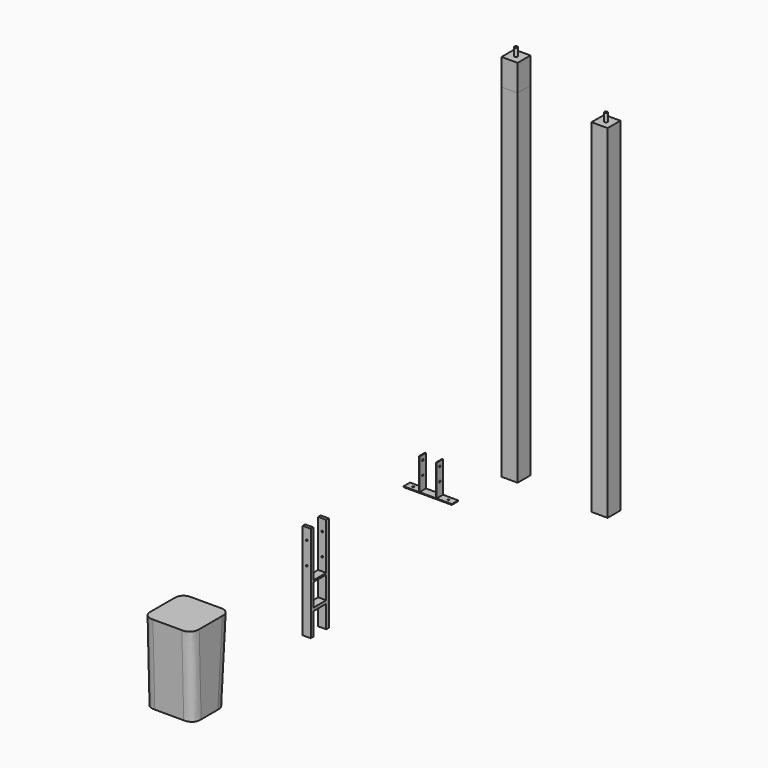
from build123d import *

# Parameters (mm, degrees)
F0_W         = 100
F0_H         = 100
F1_DEPTH     = 2300
F2_DEPTH     = 2135
F3_R         = 10
F4_DEPTH     = 50
F5_R         = 10
F6_DEPTH     = 50
F7_W         = 140
F7_H         = 600
F8_DEPTH     = 50
F9_W         = 101
F9_H         = 290.5959367752
F9_H_2       = 140
F10_DEPTH    = 100.001
F11_DEPTH    = 300
F12_T1_DEPTH = 800.2260480622
F12_T3_DEPTH = 801.2209490406
F14_W        = 300
F14_H        = 50
F15_DEPTH    = 200
F16_W        = 94.5
F16_H        = 195
F16_W_2      = 101
F17_DEPTH    = 482.3491559753
F19_D        = 10.5
F20_D        = 10.5
F21_D        = 10.5


# Not quite as in the source:
# - a fillet or chamfer that OpenCascade refuses, or shapes differently, is made with other operations: its cross-section is extruded or revolved along the edge and cut away or added


with BuildPart() as f1:
    # F0 (on Top) → F1 (new body)
    with BuildSketch(Plane.XY):
        Rectangle(F0_W, F0_H)
    extrude(amount=F1_DEPTH)

    # F3 (on face) → F4 (join)
    with BuildSketch(Plane.XY.offset(2300)):
        Circle(F3_R)
    extrude(amount=F4_DEPTH)


with BuildPart() as f2:
    # F0 (on Top) → F2 (new body)
    with BuildSketch(Plane.XY):
        Rectangle(F0_W, F0_H)
    extrude(amount=F2_DEPTH)


with BuildPart() as f2b:
    # F0 (on Top) → F2, piece 2 (new body)
    with BuildSketch(Plane.XY):
        with Locations((572.3989486694, -15.5273422599)):
            Rectangle(F0_W, F0_H)
    extrude(amount=F2_DEPTH)

    # F5 (on face) → F6 (join)
    with BuildSketch(Plane.XY.offset(2135)):
        with Locations((572.3989486694, -15.5273422599)):
            Circle(F5_R)
    extrude(amount=F6_DEPTH)


with BuildPart() as f8:
    # F7 (on Right) → F8 (new body)
    with BuildSketch(Plane.YZ):
        with Locations((-1588.707132116, 102.0108014345)):
            Rectangle(F7_W, F7_H)
    extrude(amount=F8_DEPTH)

    # F9 (on face) → F10 (cut, through all)
    with BuildSketch(Plane.YZ.offset(50)):
        with Locations((-1588.707132116, 256.7128330469)):
            Rectangle(F9_W, F9_H)
        with Locations((-1588.707132116, 31.4230661094)):
            Rectangle(F9_W, F9_H_2)
        with Locations((-1588.707132116, -127.9891985655)):
            Rectangle(F9_W, F9_H_2)
    extrude(amount=-F10_DEPTH, mode=Mode.SUBTRACT)

    # F19 (through all)
    with Locations(Plane.XZ.offset(1658.707132116)):
        with Locations((25, 330.6745588779), (25, 191.4181262255)):
            Hole(F19_D / 2)


with BuildPart() as f11:
    # F9 (on face) → F11 (new body)
    with BuildSketch(Plane.YZ.offset(50)):
        Polygon((-2661.4876322974, 454.1331665205), (-2961.4876322974, 454.1331665205), (-2946.4510382692, -45.8668334795), (-2696.4510382692, -45.8668334795), align=None)
    extrude(amount=F11_DEPTH)

    # F12: fillet of radius 60 on 4 edges, made by hand

    # F12_s2 → F12_t1 (cut)
    with BuildSketch(Plane(origin=(0, -20.8297708127, 692.6359378174), x_dir=(1, 0, 0), z_dir=(0, 0.0300595982, -0.9995481082))):
        with BuildLine():
            add(Edge.make_bspline(
                [(290, 2946.4982997158), (350, 2946.4982997158), (350, 2886.4982997158)],
                knots=[0, 0, 0, 1, 1, 1], degree=2, weights=[1, 1, 1]))
            Line((350, 2886.4982997158), (350, 2946.4982997158))
            Line((350, 2946.4982997158), (290, 2946.4982997158))
        make_face()
        with BuildLine():
            add(Edge.make_bspline(
                [(110, 2946.4982997158), (50, 2946.4982997158), (50, 2886.4982997158)],
                knots=[0, 0, 0, 1, 1, 1], degree=2, weights=[1, 1, 1]))
            Line((50, 2886.4982997158), (50, 2946.4982997158))
            Line((50, 2946.4982997158), (110, 2946.4982997158))
        make_face()
    extrude(amount=F12_T1_DEPTH, mode=Mode.SUBTRACT)

    # F12_s4 → F12_t3 (cut)
    with BuildSketch(Plane(origin=(0, -26.776023858, -382.9149808747), x_dir=(1, 0, 0), z_dir=(0, 0.0697564737, 0.9975640503))):
        with BuildLine():
            add(Edge.make_bspline(
                [(110, -2686.6831104978), (50, -2686.6831104978), (50, -2746.6831104978)],
                knots=[0, 0, 0, 1, 1, 1], degree=2, weights=[1, 1, 1]))
            Line((50, -2746.6831104978), (50, -2686.6831104978))
            Line((50, -2686.6831104978), (110, -2686.6831104978))
        make_face()
        with BuildLine():
            add(Edge.make_bspline(
                [(290, -2686.6831104978), (350, -2686.6831104978), (350, -2746.6831104978)],
                knots=[0, 0, 0, 1, 1, 1], degree=2, weights=[1, 1, 1]))
            Line((350, -2746.6831104978), (350, -2686.6831104978))
            Line((350, -2686.6831104978), (290, -2686.6831104978))
        make_face()
    extrude(amount=F12_T3_DEPTH, mode=Mode.SUBTRACT)


with BuildPart() as f15:
    # F14 (on Top) → F15 (new body)
    with BuildSketch(Plane.XY):
        with Locations((-203.6576080547, -407.3481559753)):
            Rectangle(F14_W, F14_H)
    extrude(amount=F15_DEPTH)

    # F16 (on face) → F17 (cut, through all)
    with BuildSketch(Plane.XZ.offset(432.3481559753)):
        with Locations((-306.4076080547, 102.5)):
            Rectangle(F16_W, F16_H)
        with Locations((-203.6576080547, 102.5)):
            Rectangle(F16_W_2, F16_H)
        with Locations((-100.9076080547, 102.5)):
            Rectangle(F16_W, F16_H)
    extrude(amount=-F17_DEPTH, mode=Mode.SUBTRACT)

    # F20 (through all)
    with Locations(Plane(origin=(0, 0, 0), x_dir=(1, 0, 0), z_dir=(0, 0, -1))):
        with Locations((-313.6576080547, 407.3481559753), (-93.6576080547, 407.3481559753)):
            Hole(F20_D / 2)

    # F21 (through all)
    with Locations(Plane(origin=(-259.1576080547, 0, 0), x_dir=(0, -1, 0), z_dir=(-1, 0, 0))):
        with Locations((407.3481559753, 170.6195473671), (407.3481559753, 87.6534283161)):
            Hole(F21_D / 2)


solid = Compound([f1.part, f2.part, f2b.part, f8.part, f11.part, f15.part])
